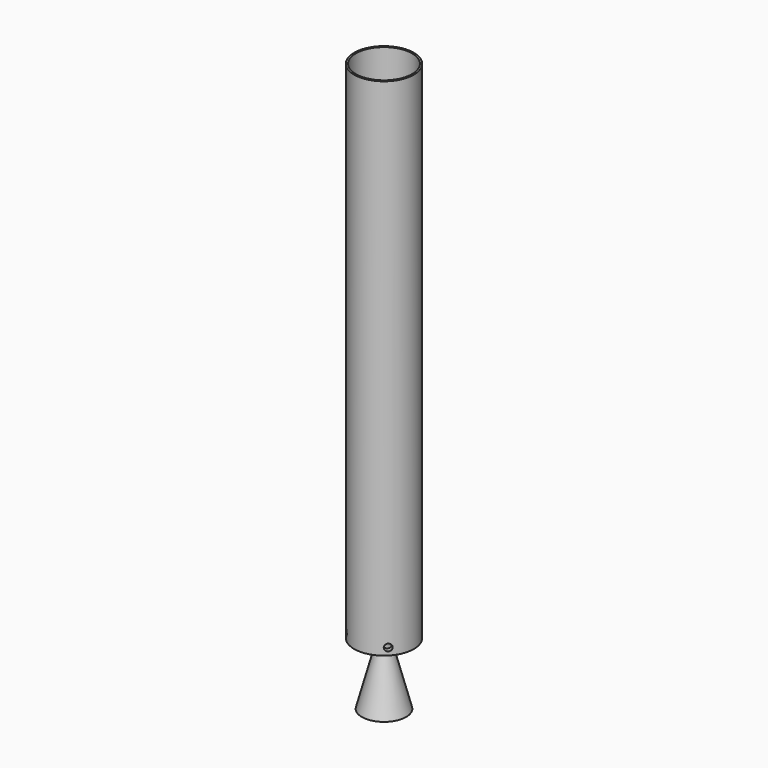
from build123d import *

# Parameters (mm, degrees)
F6_R      = 3.175
F7_DEPTH  = 25.4
F9_R      = 3.175
F10_DEPTH = 25.4
F11_DEPTH = 25.4
F13_R     = 3.175
F14_DEPTH = 25.4
F16_R     = 3.175
F17_DEPTH = 25.4
F18_ANGLE = 45


with BuildPart() as f1:
    # F0 (on Front) → F1 (revolve)
    with BuildSketch(Plane.XZ):
        with BuildLine():
            Line((-5.4717690375, -28.4604633269), (-25.4, 0))
            Line((-25.4, 0), (-25.4, -31.75))
            Line((-25.4, -31.75), (-22.225, -31.75))
            Line((-22.225, -31.75), (-22.225, -10.0698134975))
            Line((-22.225, -10.0698134975), (-8.0725767781, -30.2815685124))
            ThreePointArc((-8.0725767781, -30.2815685124), (-6.4947061526, -34.0908851763), (-6.6745565046, -38.2101354732))
            Line((-6.6745565046, -38.2101354732), (-20.0427513701, -88.1009179169))
            Line((-20.0427513701, -88.1009179169), (-16.7557494973, -88.1009179169))
            Line((-16.7557494973, -88.1009179169), (-3.6077420061, -39.0318859414))
            ThreePointArc((-3.6077420061, -39.0318859414), (-3.3679415367, -33.5395522122), (-5.4717690375, -28.4604633269))
        make_face()
    revolve(axis=Axis((0, 0, -44.0504589584), (0, 0, -1)))


with BuildPart() as f3:
    # F2 (on Front) → F3 (revolve)
    with BuildSketch(Plane.XZ):
        Polygon((26.9875, 457.2), (25.4, 457.2), (25.4, 355.6), (0, 355.6), (0, 352.425), (25.4, 352.425), (25.4, 0), (26.9875, 0), align=None)
    revolve(axis=Axis((0, 0, 228.6), (0, 0, 1)))


with BuildPart() as f1_1:
    # F4: moved
    add(f1.part.moved(Location((0, 0, 31.75))))


with BuildPart() as f7_tool:
    # F6 (on offset) → F7 (new body)
    with BuildSketch(Plane.YZ.offset(20.32)):
        with Locations((0, 6.35)):
            Circle(F6_R)
    extrude(amount=F7_DEPTH)


with BuildPart() as f1_2:
    add(f1_1.part)

    # F7: cut by f7_tool
    add(f7_tool.part, mode=Mode.SUBTRACT)


with BuildPart() as f3_1:
    add(f3.part)

    # F7: cut by f7_tool
    add(f7_tool.part, mode=Mode.SUBTRACT)


with BuildPart() as f10_tool:
    # F9 (on offset) → F10 (new body)
    with BuildSketch(Plane.YZ.offset(-20.32)):
        with Locations((0, 6.35)):
            Circle(F9_R)
    extrude(amount=-F10_DEPTH)


with BuildPart() as f1_3:
    add(f1_2.part)

    # F10: cut by f10_tool
    add(f10_tool.part, mode=Mode.SUBTRACT)

    # F6 (on offset) → F11 (cut)
    with BuildSketch(Plane.YZ.offset(20.32)):
        with Locations((0, 6.35)):
            Circle(F6_R)
    extrude(amount=F11_DEPTH, mode=Mode.SUBTRACT)


with BuildPart() as f3_2:
    add(f3_1.part)

    # F10: cut by f10_tool
    add(f10_tool.part, mode=Mode.SUBTRACT)


with BuildPart() as f14_tool:
    # F13 (on offset) → F14 (new body)
    with BuildSketch(Plane.XZ.offset(20.32)):
        with Locations((0, 6.35)):
            Circle(F13_R)
    extrude(amount=F14_DEPTH)


with BuildPart() as f1_4:
    add(f1_3.part)

    # F14: cut by f14_tool
    add(f14_tool.part, mode=Mode.SUBTRACT)


with BuildPart() as f3_3:
    add(f3_2.part)

    # F14: cut by f14_tool
    add(f14_tool.part, mode=Mode.SUBTRACT)


with BuildPart() as f17_tool:
    # F16 (on offset) → F17 (new body)
    with BuildSketch(Plane.XZ.offset(-20.32)):
        with Locations((0, 6.35)):
            Circle(F16_R)
    extrude(amount=-F17_DEPTH)


with BuildPart() as f1_5:
    add(f1_4.part)

    # F17: cut by f17_tool
    add(f17_tool.part, mode=Mode.SUBTRACT)


with BuildPart() as f3_4:
    add(f3_3.part)

    # F17: cut by f17_tool
    add(f17_tool.part, mode=Mode.SUBTRACT)


with BuildPart() as f1_6:
    # F18: moved
    add(f1_5.part.rotate(Axis((0, 0, 457.2), (0, 0, 1)), F18_ANGLE))


with BuildPart() as f3_5:
    # F18: moved
    add(f3_4.part.rotate(Axis((0, 0, 457.2), (0, 0, 1)), F18_ANGLE))


solid = Compound([f1_6.part, f3_5.part])
